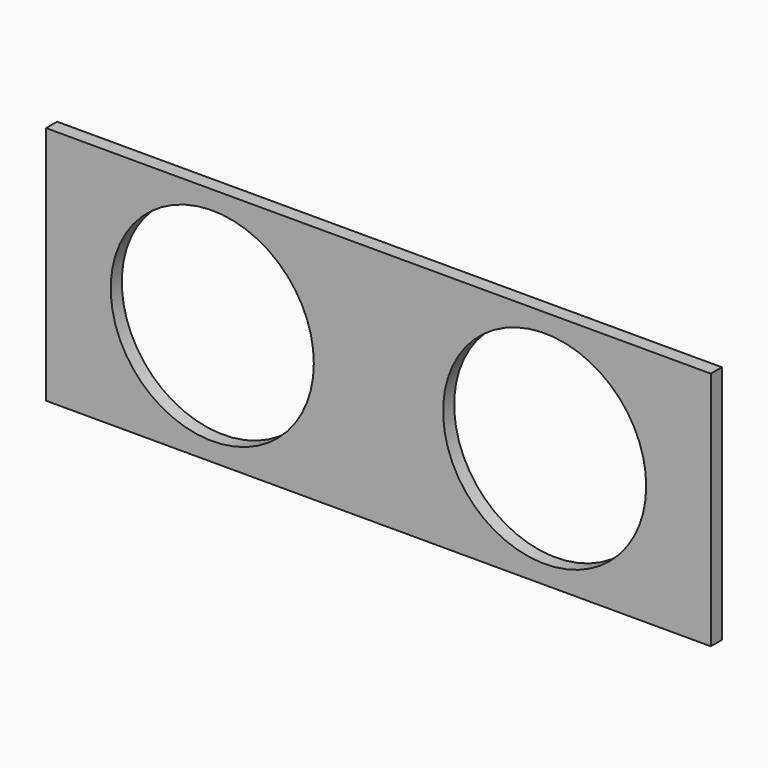
from build123d import *

# Parameters (mm, degrees)
F0_W     = 914.4
F0_H     = 330.2
F2_DEPTH = 19.05
F1_R     = 139.7
F3_DEPTH = 982
F4_DEPTH = 19.051
F5_R     = 139.7
F6_DEPTH = 19.051


# Not quite as in the source:
# - an extrude ends at something that could not be found from the text; its depth is read off the source's solid


with BuildPart() as f2:
    # F0 (on Front) → F2 (new body)
    with BuildSketch(Plane.XZ):
        Rectangle(F0_W, F0_H)
    extrude(amount=F2_DEPTH)

    # F1 (on face) → F3 (cut, through all)
    with BuildSketch(Plane.XZ):
        with Locations((-228.6, 0)):
            Circle(F1_R)
    extrude(amount=-F3_DEPTH, mode=Mode.SUBTRACT)

    # F1 (on face) → F4 (cut, through all)
    with BuildSketch(Plane.XZ):
        with Locations((-228.6, 0)):
            Circle(F1_R)
    extrude(amount=F4_DEPTH, mode=Mode.SUBTRACT)

    # F5 (on face) → F6 (cut, through all)
    with BuildSketch(Plane.XZ.offset(19.05)):
        with Locations((228.6, 0)):
            Circle(F5_R)
    extrude(amount=-F6_DEPTH, mode=Mode.SUBTRACT)


solid = f2.part
